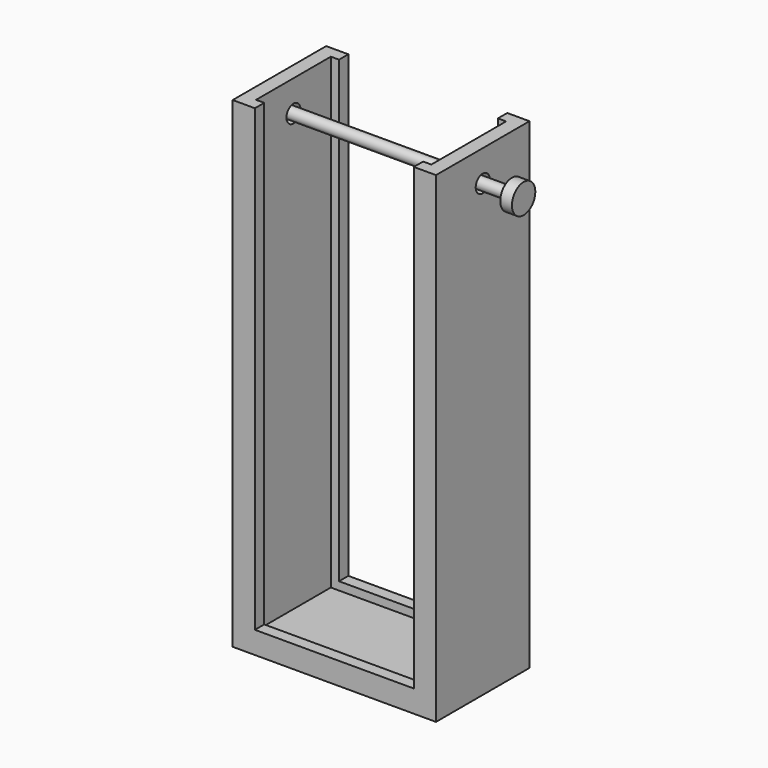
from build123d import *

# Parameters (mm, degrees)
F1_DEPTH      = 4
F1_DEPTH_BACK = 4
F2_START      = -4
F2_DEPTH      = 1
F3_START      = 4
F3_DEPTH      = 1
F4_R          = 0.75
F4_R_2        = 0.5
F5_DEPTH      = 25
F6_DEPTH      = 2.5
F6_DEPTH_BACK = 19.9
F7_START      = 2.5
F4_R_3        = 1.25
F7_DEPTH      = 1


# Not quite as in the source:
# - a feature names something its author has since deleted; it is built from what else it names


with BuildPart() as f1:
    # F0 (on Front) → F1 (new body, two sides)
    with BuildSketch(Plane.XZ) as f1_sk:
        Polygon((7.5, 20), (7.5, -20), (-7.5, -20), (-7.5, 20), (-8.7, 20), (-8.7, -21.2), (8.7, -21.2), (8.7, 20), align=None)
    extrude(amount=F1_DEPTH)
    extrude(f1_sk.sketch, amount=-F1_DEPTH_BACK)

    # F0 (on Front) → F2 (join)
    with BuildSketch(Plane.XZ.offset(F2_START)):
        Polygon((-7.5, -20), (7.5, -20), (7.5, 20), (6.8, 20), (6.8, -19.3), (-6.8, -19.3), (-6.8, 20), (-7.5, 20), align=None)
        Polygon((7.5, 20), (7.5, -20), (-7.5, -20), (-7.5, 20), (-8.7, 20), (-8.7, -21.2), (8.7, -21.2), (8.7, 20), align=None)
    extrude(amount=-F2_DEPTH)

    # F0 (on Front) → F3 (join)
    with BuildSketch(Plane.XZ.offset(F3_START)):
        Polygon((7.5, 20), (7.5, -20), (-7.5, -20), (-7.5, 20), (-8.7, 20), (-8.7, -21.2), (8.7, -21.2), (8.7, 20), align=None)
        Polygon((-7.5, -20), (7.5, -20), (7.5, 20), (6.8, 20), (6.8, -19.3), (-6.8, -19.3), (-6.8, 20), (-7.5, 20), align=None)
    extrude(amount=F3_DEPTH)

    # F4 (on face) → F5 (cut)
    with BuildSketch(Plane.YZ.offset(8.7)):
        with Locations((0, 17.3376215611)):
            Circle(F4_R)
        with Locations((0, 17.3376215611)):
            Circle(F4_R_2, mode=Mode.SUBTRACT)
    extrude(amount=-F5_DEPTH, mode=Mode.SUBTRACT)


with BuildPart() as f6:
    # F4 (on face) → F6 (new body, two sides)
    with BuildSketch(Plane.YZ.offset(8.7)) as f6_sk:
        with Locations((0, 17.3376215611)):
            Circle(F4_R_2)
    extrude(amount=F6_DEPTH)
    extrude(f6_sk.sketch, amount=-F6_DEPTH_BACK)

    # F4 (on face) → F7 (join)
    with BuildSketch(Plane.YZ.offset(8.7).offset(F7_START)):
        with Locations((0, 17.3376215611)):
            Circle(F4_R_3)
        with Locations((0, 17.3376215611)):
            Circle(F4_R, mode=Mode.SUBTRACT)
        with Locations((0, 17.3376215611)):
            Circle(F4_R)
        with Locations((0, 17.3376215611)):
            Circle(F4_R_2, mode=Mode.SUBTRACT)
        with Locations((0, 17.3376215611)):
            Circle(F4_R_2)
    extrude(amount=F7_DEPTH)


solid = Compound([f1.part, f6.part])
